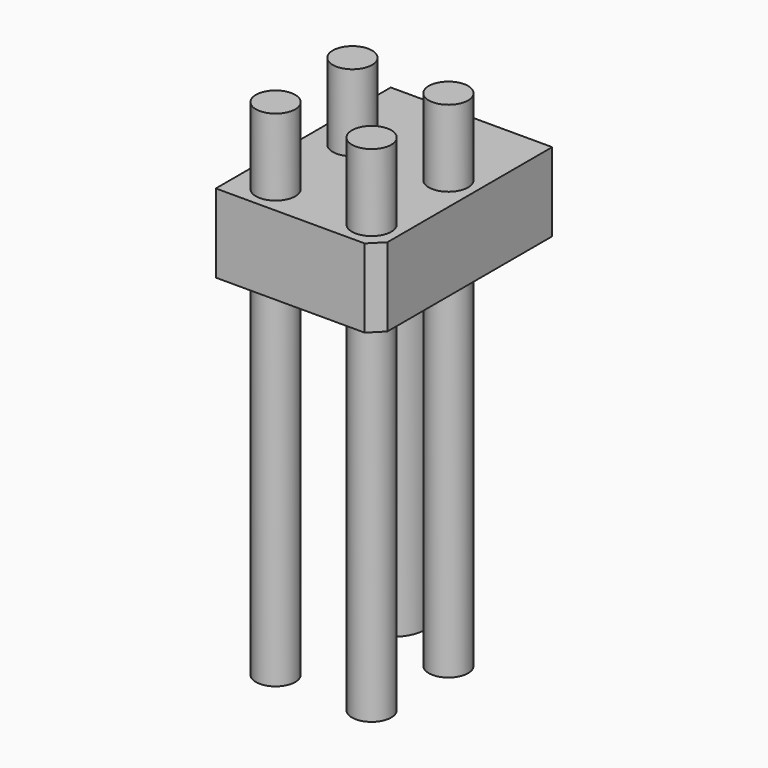
from build123d import *

# Parameters (mm, degrees)
F1_DEPTH = 900
F2_R     = 450
F3_DEPTH = 1755
F4_R     = 450
F4_R_2   = 750
F5_DEPTH = 8000


# Not quite as in the source:
# - the program builds the solid bodies; features that only make, move or delete a surface that nothing else refers to are left out


with BuildPart() as f1:
    # F0 (on Top) → F1 (new body, symmetric)
    with BuildSketch(Plane.XY):
        Polygon((3604.9533605576, 6359.4330211878), (-95.0466394424, 6359.4330211878), (-95.0466394424, 1349.4330211878), (3316.1160576543, 1349.4330211878), (3604.9533605576, 1638.270324091), align=None)
    extrude(amount=F1_DEPTH, both=True)

    # F2 (on face) → F3 (join)
    with BuildSketch(Plane.XY.offset(900)):
        with Locations((754.9533605576, 4199.4330211878)):
            Circle(F2_R)
        with Locations((754.9533605576, 1999.4330211878)):
            Circle(F2_R)
        with Locations((2954.9533605576, 4199.4330211878)):
            Circle(F2_R)
        with Locations((2954.9533605576, 1999.4330211878)):
            Circle(F2_R)
    extrude(amount=F3_DEPTH)

    # F4 (on face) → F5 (join)
    with BuildSketch(Plane(origin=(0, 0, -900), x_dir=(1, 0, 0), z_dir=(0, 0, -1))):
        with Locations((754.9533605576, -1999.4330211878)):
            Circle(F4_R)
        with Locations((2954.9533605576, -1999.4330211878)):
            Circle(F4_R)
        with Locations((2954.9533605576, -4199.4330211878)):
            Circle(F4_R)
        with Locations((1004.9533605576, -5045.4330211878)):
            Circle(F4_R_2)
    extrude(amount=F5_DEPTH)


solid = f1.part
